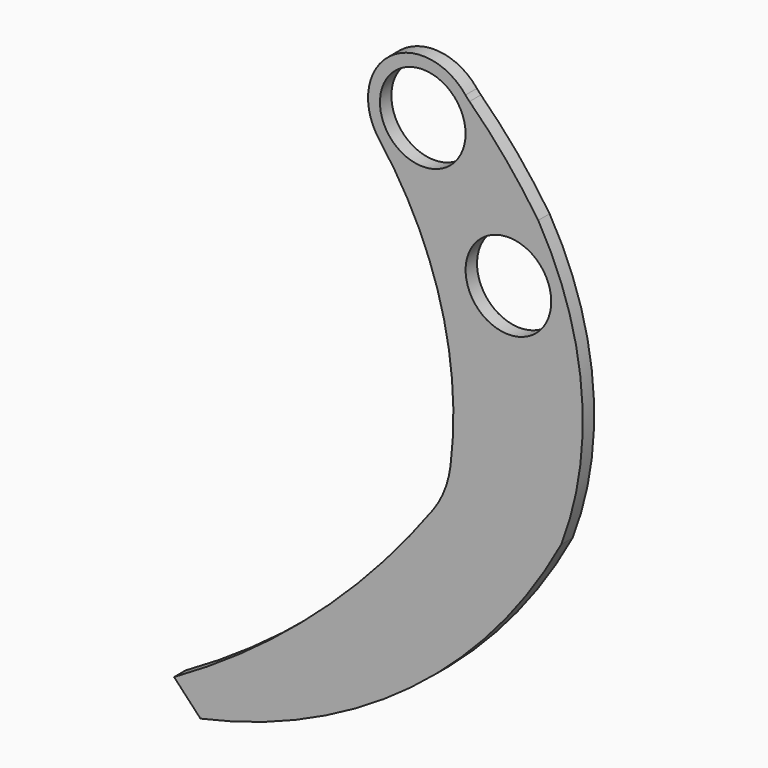
from build123d import *

# Parameters (mm, degrees)
F0_R     = 45
F1_DEPTH = 15


# Not quite as in the source:
# - ends of sketch curves that miss each other by under 0.0002 mm in the source are joined


with BuildPart() as f1:
    # F0 (on Front) → F1 (new body)
    with BuildSketch(Plane.XZ):
        with BuildLine():
            Line((508.886889, 467.23394), (536.629649, 437.761061))
            ThreePointArc((536.629649, 437.761061), (757.5121515647, 538.3707556644), (915.8713779319, 722.3102730367))
            ThreePointArc((915.8713779319, 722.3102730367), (937.3750069367, 871.1241026292), (891.6662720762, 1014.3675090452))
            ThreePointArc((891.6662720762, 1014.3675090452), (857.8155387776, 1059.5076628094), (819.4482445104, 1100.877414496))
            ThreePointArc((819.4482445104, 1100.877414496), (817.2633574779, 1103.137500552), (815.2248101142, 1105.5304160912))
            ThreePointArc((815.2248101142, 1105.5304160912), (734.7474434458, 1114.8247485045), (724.8508240235, 1034.4192260182))
            ThreePointArc((724.8508240235, 1034.4192260182), (789.4425603105, 903.419496525), (799.5567075135, 757.7118249354))
            ThreePointArc((799.5567075135, 757.7118249354), (793.3301361175, 732.8130625575), (780.9710848276, 710.319232126))
            ThreePointArc((780.9710848276, 710.319232126), (657.7707545167, 574.4028574869), (508.886889, 467.23394))
        make_face()
        with Locations((860.37194, 943.574077)):
            Circle(F0_R, mode=Mode.SUBTRACT)
        with Locations((770.304035, 1069.636489)):
            Circle(F0_R, mode=Mode.SUBTRACT)
    extrude(amount=F1_DEPTH)


solid = f1.part
